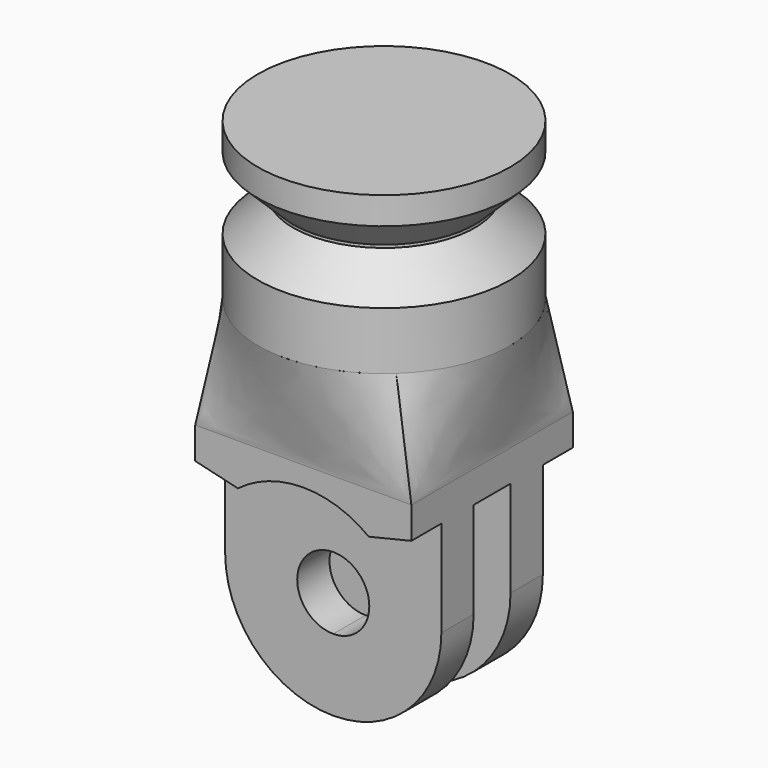
from build123d import *

# Parameters (mm, degrees)
F1_START  = 1.6
F1_DEPTH  = 2.8
F2_DEPTH  = 7
F3_FACE_W = 15
F3_FACE_H = 14


# Not quite as in the source:
# - the arcs of a loft's sections are written as splines that run evenly, so that the points pair up as in the source's solid


with BuildPart() as f1:
    # F0 (on Front) → F1 (new body)
    with BuildSketch(Plane.XZ.offset(F1_START)):
        with BuildLine():
            ThreePointArc((4.5405321415, 5.9693858873), (6.7195234601, 3.331366757), (7.5, 0))
            Line((7.5, 0), (7.5, 6.6765861305))
            Line((7.5, 6.6765861305), (4.5405321415, 5.9693858873))
        make_face()
        with BuildLine():
            Line((-7.5, 6.6765861305), (-7.5, 0))
            ThreePointArc((-7.5, 0), (-6.7195234601, 3.331366757), (-4.5405321415, 5.9693858873))
            Line((-4.5405321415, 5.9693858873), (-7.5, 6.6765861305))
        make_face()
        with BuildLine():
            ThreePointArc((0, 7.5), (2.3957885805, 7.1070526294), (4.5405321415, 5.9693858873))
            Line((4.5405321415, 5.9693858873), (7.5, 6.6765861305))
            Line((7.5, 6.6765861305), (7.5, 8.8696251196))
            Line((7.5, 8.8696251196), (0, 8.8696251196))
            Line((0, 8.8696251196), (0, 7.5))
        make_face()
        with BuildLine():
            ThreePointArc((-4.5405321415, 5.9693858873), (-2.3957885805, 7.1070526294), (0, 7.5))
            Line((0, 7.5), (0, 8.8696251196))
            Line((0, 8.8696251196), (-7.5, 8.8696251196))
            Line((-7.5, 8.8696251196), (-7.5, 6.6765861305))
            Line((-7.5, 6.6765861305), (-4.5405321415, 5.9693858873))
        make_face()
        with BuildLine():
            ThreePointArc((0, -7.5), (5.3033008589, -5.3033008589), (7.5, 0))
            ThreePointArc((7.5, 0), (6.7195234601, 3.331366757), (4.5405321415, 5.9693858873))
            ThreePointArc((4.5405321415, 5.9693858873), (2.3957885805, 7.1070526294), (0, 7.5))
            Line((0, 7.5), (0, 2.5))
            ThreePointArc((0, 2.5), (1.767766953, 1.767766953), (2.5, 0))
            ThreePointArc((2.5, 0), (1.767766953, -1.767766953), (0, -2.5))
            Line((0, -2.5), (0, -7.5))
        make_face()
        with BuildLine():
            ThreePointArc((-7.5, 0), (-5.3033008589, -5.3033008589), (0, -7.5))
            Line((0, -7.5), (0, -2.5))
            ThreePointArc((0, -2.5), (-2.5, 0), (0, 2.5))
            Line((0, 2.5), (0, 7.5))
            ThreePointArc((0, 7.5), (-2.3957885805, 7.1070526294), (-4.5405321415, 5.9693858873))
            ThreePointArc((-4.5405321415, 5.9693858873), (-6.7195234601, 3.331366757), (-7.5, 0))
        make_face()
    extrude(amount=F1_DEPTH)

    # F0 (on Front) → F2 (join)
    with BuildSketch(Plane.XZ):
        with BuildLine():
            ThreePointArc((-4.5405321415, 5.9693858873), (-2.3957885805, 7.1070526294), (0, 7.5))
            Line((0, 7.5), (0, 8.8696251196))
            Line((0, 8.8696251196), (-7.5, 8.8696251196))
            Line((-7.5, 8.8696251196), (-7.5, 6.6765861305))
            Line((-7.5, 6.6765861305), (-4.5405321415, 5.9693858873))
        make_face()
        with BuildLine():
            ThreePointArc((0, 7.5), (2.3957885805, 7.1070526294), (4.5405321415, 5.9693858873))
            Line((4.5405321415, 5.9693858873), (7.5, 6.6765861305))
            Line((7.5, 6.6765861305), (7.5, 8.8696251196))
            Line((7.5, 8.8696251196), (0, 8.8696251196))
            Line((0, 8.8696251196), (0, 7.5))
        make_face()
    extrude(amount=F2_DEPTH)

    # F3: F1 across face


with BuildPart() as f1_1:
    add(f1.part)
    add(f1.part.mirror(Plane(origin=(0, 0, 7.7459450352), x_dir=(1, 0, 0), z_dir=(0, 1, 0))))



with BuildPart() as f4:
    # F0 (on Front) → F4 (revolve)
    with BuildSketch(Plane.XZ):
        Polygon((-8.75, 16.1584225655), (0, 16.1584225655), (0, 27.0584225655), (-8.75, 27.0584225655), (-8.75, 25.1584225655), (-6.3, 22.7584225655), (-6.3, 22.5584225655), (-8.75, 20.1584225655), align=None)
    revolve(axis=Axis((0, 0, 25.701952844), (0, 0, 1)))


with BuildPart() as f1_2:
    add(f1_1.part)

    add(f4.part)  # F5 merges F4
    # F4_face (on face) → F5 section 0
    with BuildSketch(Plane(origin=(0, 0, 16.1584225655), x_dir=(1, 0, 0), z_dir=(0, 0, -1))):
        with BuildLine():
            add(Edge.make_bspline(
                [(-6.3967335971, 5.9702846907), (-7.1782420356, 5.1329542208), (-7.7929531303, 4.1405626748), (-8.5961274355, 1.9952370454), (-8.7842746312, 0.8431470561), (-8.7053303575, -1.4462368833), (-8.4382699492, -2.5826300587), (-7.4892256465, -4.6675343567), (-6.8076151605, -5.6152251586), (-5.9702846907, -6.3967335971)],
                knots=[0, 0, 0, 0, 0.25, 0.25, 0.5, 0.5, 0.75, 0.75, 1, 1, 1, 1], degree=3))
            add(Edge.make_bspline(
                [(-5.9702846907, -6.3967335971), (-5.1329542208, -7.1782420356), (-4.1405626748, -7.7929531303), (-1.9952370454, -8.5961274355), (-0.8431470561, -8.7842746312), (1.4462368833, -8.7053303575), (2.5826300587, -8.4382699492), (4.6675343567, -7.4892256465), (5.6152251586, -6.8076151605), (6.3967335971, -5.9702846907)],
                knots=[0, 0, 0, 0, 0.25, 0.25, 0.5, 0.5, 0.75, 0.75, 1, 1, 1, 1], degree=3))
            add(Edge.make_bspline(
                [(6.3967335971, -5.9702846907), (7.1782420356, -5.1329542208), (7.7929531303, -4.1405626748), (8.5961274355, -1.9952370454), (8.7842746312, -0.8431470561), (8.7053303575, 1.4462368833), (8.4382699492, 2.5826300587), (7.4892256465, 4.6675343567), (6.8076151605, 5.6152251586), (5.9702846907, 6.3967335971)],
                knots=[0, 0, 0, 0, 0.25, 0.25, 0.5, 0.5, 0.75, 0.75, 1, 1, 1, 1], degree=3))
            add(Edge.make_bspline(
                [(5.9702846907, 6.3967335971), (5.1329542208, 7.1782420356), (4.1405626748, 7.7929531303), (1.9952370454, 8.5961274355), (0.8431470561, 8.7842746312), (-1.4462368833, 8.7053303575), (-2.5826300587, 8.4382699492), (-4.6675343567, 7.4892256465), (-5.6152251586, 6.8076151605), (-6.3967335971, 5.9702846907)],
                knots=[0, 0, 0, 0, 0.25, 0.25, 0.5, 0.5, 0.75, 0.75, 1, 1, 1, 1], degree=3))
        make_face()
    # F3_face (on face) → F5 section 1
    with BuildSketch(Plane.XY.offset(8.8696251196)):
        Rectangle(F3_FACE_W, F3_FACE_H)
    loft(ruled=True)


solid = f1_2.part
